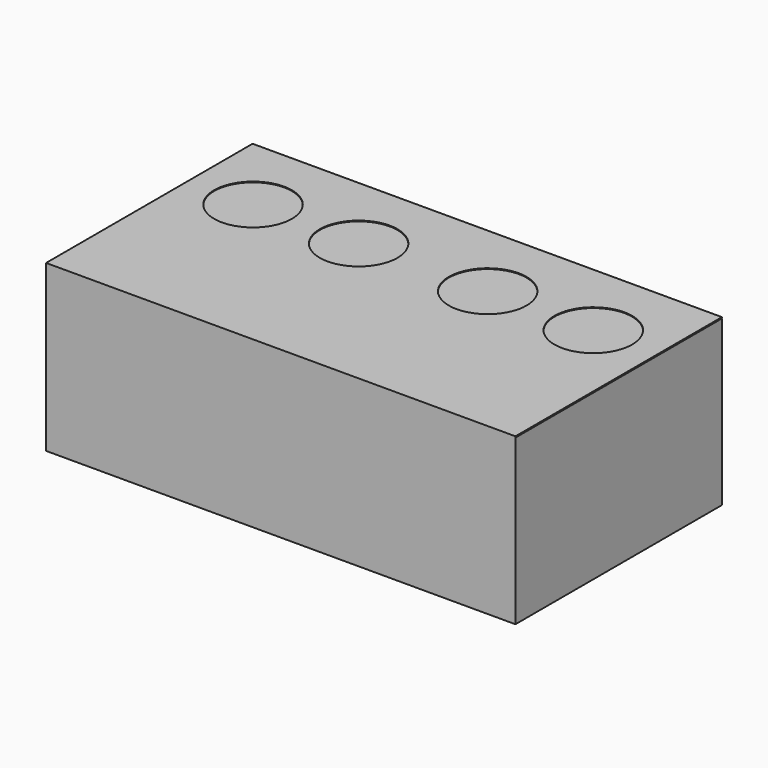
from build123d import *

# Parameters (mm, degrees)
F1_DEPTH = 127
F3_DEPTH = 0.4064


# Not quite as in the source:
# - the dataset's text gives a spline's control points without its knots; the knots are read off the source's solid


with BuildPart() as f1:
    # F0 (on Right) → F1 (new body, symmetric)
    with BuildSketch(Plane.YZ):
        Polygon((-139.7, 0), (0, 0), (0, 88.9), (-139.2936, 88.9), (-139.2936, 89.154), (0, 89.154), (0, 89.5604), (-139.7, 89.5604), align=None)
    extrude(amount=F1_DEPTH, both=True)

    # F2 (on face) → F3 (cut, through all)
    with BuildSketch(Plane.XY.offset(89.5604)):
        with BuildLine():
            add(Edge.make_bspline(
                [(-20.0838931644, -58.1858374521), (-16.1902509644, -54.2918904521), (-13.9233771644, -48.8190032521), (-13.9233771644, -43.3123340521), (-13.9233771644, -37.8053854521), (-16.1902509644, -32.3324982521), (-20.0838931644, -28.4388560521), (-23.9778909644, -24.5448582521), (-29.4507781644, -22.2779590521), (-34.9577521644, -22.2779590521)],
                knots=[5, 5, 5, 5, 6, 6, 6, 7, 7, 7, 8, 8, 8, 8], degree=3))
            add(Edge.make_bspline(
                [(-34.9577521644, -22.2779590521), (-40.4643959644, -22.2779590521), (-45.9372831644, -24.5448582521), (-49.8309253644, -28.4388560521)],
                knots=[0, 0, 0, 0, 1, 1, 1, 1], degree=3))
            add(Edge.make_bspline(
                [(-49.8309253644, -28.4388560521), (-53.7249231644, -32.3324982521), (-55.9921271644, -37.8053854521), (-55.9921271644, -43.3123340521), (-55.9921271644, -48.8190032521), (-53.7249231644, -54.2918904521), (-49.8309253644, -58.1858374521)],
                knots=[1, 1, 1, 1, 2, 2, 2, 3, 3, 3, 3], degree=3))
            add(Edge.make_bspline(
                [(-49.8309253644, -58.1858374521), (-45.9372831644, -62.0795304521), (-40.4643959644, -64.3467090521), (-34.9577521644, -64.3467090521), (-29.4507781644, -64.3467090521), (-23.9778909644, -62.0795304521), (-20.0838931644, -58.1858374521)],
                knots=[3, 3, 3, 3, 4, 4, 4, 5, 5, 5, 5], degree=3))
        make_face()
        with BuildLine():
            add(Edge.make_bspline(
                [(49.7661068356, -58.1858374521), (53.6597490356, -54.2918904521), (55.9266228356, -48.8190032521), (55.9266228356, -43.3123340521), (55.9266228356, -37.8053854521), (53.6597490356, -32.3324982521), (49.7661068356, -28.4388560521), (45.8721090356, -24.5448582521), (40.3992218356, -22.2779590521), (34.8922478356, -22.2779590521)],
                knots=[5, 5, 5, 5, 6, 6, 6, 7, 7, 7, 8, 8, 8, 8], degree=3))
            add(Edge.make_bspline(
                [(34.8922478356, -22.2779590521), (29.3856040356, -22.2779590521), (23.9127168356, -24.5448582521), (20.0190746356, -28.4388560521)],
                knots=[0, 0, 0, 0, 1, 1, 1, 1], degree=3))
            add(Edge.make_bspline(
                [(20.0190746356, -28.4388560521), (16.1250768356, -32.3324982521), (13.8578728356, -37.8053854521), (13.8578728356, -43.3123340521), (13.8578728356, -48.8190032521), (16.1250768356, -54.2918904521), (20.0190746356, -58.1858374521)],
                knots=[1, 1, 1, 1, 2, 2, 2, 3, 3, 3, 3], degree=3))
            add(Edge.make_bspline(
                [(20.0190746356, -58.1858374521), (23.9127168356, -62.0795304521), (29.3856040356, -64.3467090521), (34.8922478356, -64.3467090521), (40.3992218356, -64.3467090521), (45.8721090356, -62.0795304521), (49.7661068356, -58.1858374521)],
                knots=[3, 3, 3, 3, 4, 4, 4, 5, 5, 5, 5], degree=3))
        make_face()
        with BuildLine():
            add(Edge.make_bspline(
                [(106.9161068356, -58.1858374521), (110.8097490356, -54.2918904521), (113.0766228356, -48.8190032521), (113.0766228356, -43.3123340521), (113.0766228356, -37.8053854521), (110.8097490356, -32.3324982521), (106.9161068356, -28.4388560521), (103.0221090356, -24.5448582521), (97.5492218356, -22.2779590521), (92.0422478356, -22.2779590521)],
                knots=[5, 5, 5, 5, 6, 6, 6, 7, 7, 7, 8, 8, 8, 8], degree=3))
            add(Edge.make_bspline(
                [(92.0422478356, -22.2779590521), (86.5356040356, -22.2779590521), (81.0627168356, -24.5448582521), (77.1690746356, -28.4388560521)],
                knots=[0, 0, 0, 0, 1, 1, 1, 1], degree=3))
            add(Edge.make_bspline(
                [(77.1690746356, -28.4388560521), (73.2750768356, -32.3324982521), (71.0078728356, -37.8053854521), (71.0078728356, -43.3123340521), (71.0078728356, -48.8190032521), (73.2750768356, -54.2918904521), (77.1690746356, -58.1858374521)],
                knots=[1, 1, 1, 1, 2, 2, 2, 3, 3, 3, 3], degree=3))
            add(Edge.make_bspline(
                [(77.1690746356, -58.1858374521), (81.0627168356, -62.0795304521), (86.5356040356, -64.3467090521), (92.0422478356, -64.3467090521), (97.5492218356, -64.3467090521), (103.0221090356, -62.0795304521), (106.9161068356, -58.1858374521)],
                knots=[3, 3, 3, 3, 4, 4, 4, 5, 5, 5, 5], degree=3))
        make_face()
        with BuildLine():
            add(Edge.make_bspline(
                [(-77.2338931644, -58.1858374521), (-73.3402509644, -54.2918904521), (-71.0733771644, -48.8190032521), (-71.0733771644, -43.3123340521), (-71.0733771644, -37.8053854521), (-73.3402509644, -32.3324982521), (-77.2338931644, -28.4388560521), (-81.1278909644, -24.5448582521), (-86.6007781644, -22.2779590521), (-92.1077521644, -22.2779590521)],
                knots=[5, 5, 5, 5, 6, 6, 6, 7, 7, 7, 8, 8, 8, 8], degree=3))
            add(Edge.make_bspline(
                [(-92.1077521644, -22.2779590521), (-97.6143959644, -22.2779590521), (-103.0872831644, -24.5448582521), (-106.9812301644, -28.4388560521)],
                knots=[0, 0, 0, 0, 1, 1, 1, 1], degree=3))
            add(Edge.make_bspline(
                [(-106.9812301644, -28.4388560521), (-110.8749231644, -32.3324982521), (-113.1421271644, -37.8053854521), (-113.1421271644, -43.3123340521), (-113.1421271644, -48.8190032521), (-110.8749231644, -54.2918904521), (-106.9812301644, -58.1858374521)],
                knots=[1, 1, 1, 1, 2, 2, 2, 3, 3, 3, 3], degree=3))
            add(Edge.make_bspline(
                [(-106.9812301644, -58.1858374521), (-103.0872831644, -62.0795304521), (-97.6143959644, -64.3467090521), (-92.1077521644, -64.3467090521), (-86.6007781644, -64.3467090521), (-81.1278909644, -62.0795304521), (-77.2338931644, -58.1858374521)],
                knots=[3, 3, 3, 3, 4, 4, 4, 5, 5, 5, 5], degree=3))
        make_face()
    extrude(amount=-F3_DEPTH, mode=Mode.SUBTRACT)


solid = f1.part
